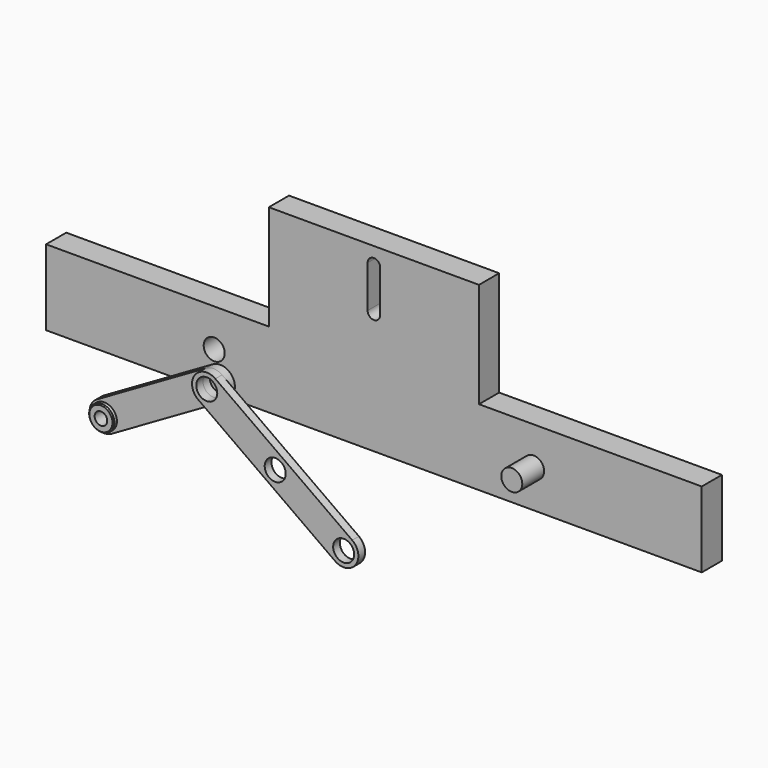
from build123d import *

# Parameters (mm, degrees)
F0_W      = 156
F0_H      = 6
F1_DEPTH  = 9
F2_R      = 2.5
F3_DEPTH  = 6
F5_R      = 2.5
F6_DEPTH  = 7
F7_R      = 2
F8_DEPTH  = 5
F9_R      = 2.5
F10_DEPTH = 6.5
F11_W     = 50
F11_H     = 6
F12_DEPTH = 25
F14_DEPTH = 6
F15_R     = 2.5
F16_DEPTH = 2
F17_R     = 2.5
F18_DEPTH = 2
F20_R     = 2.5
F21_DEPTH = 2.1
F22_R     = 3
F23_DEPTH = 1
F24_R     = 1.5
F25_DEPTH = 3.1
F26_SIZE  = 0.25


with BuildPart() as f1:
    # F0 (on Top) → F1 (new body, symmetric)
    with BuildSketch(Plane.XY):
        with Locations((0, -38.5)):
            Rectangle(F0_W, F0_H)
    extrude(amount=F1_DEPTH, both=True)

    # F2 (on face) → F3 (cut, through all)
    with BuildSketch(Plane.XZ.offset(41.5)):
        with Locations((-38, 0)):
            Circle(F2_R)
        with Locations((38, 0)):
            Circle(F2_R)
    extrude(amount=-F3_DEPTH, mode=Mode.SUBTRACT)

    # F11 (on face) → F12 (join)
    with BuildSketch(Plane.XY.offset(9)):
        with Locations((0, -38.5)):
            Rectangle(F11_W, F11_H)
    extrude(amount=F12_DEPTH)

    # F13 (on face) → F14 (cut, through all)
    with BuildSketch(Plane.XZ.offset(41.5)):
        with BuildLine():
            ThreePointArc((1.5, 30), (0, 31.5), (-1.5, 30))
            Line((-1.5, 30), (-1.5, 20))
            ThreePointArc((-1.5, 20), (0, 18.5), (1.5, 20))
            Line((1.5, 20), (1.5, 30))
        make_face()
    extrude(amount=-F14_DEPTH, mode=Mode.SUBTRACT)


with BuildPart() as f6:
    # F5 (on face) → F6 (new body)
    with BuildSketch(Plane.XZ.offset(41.5)):
        with Locations((38, 0)):
            Circle(F5_R)
    extrude(amount=-F6_DEPTH)

    # F7 (on face) → F8 (join)
    with BuildSketch(Plane(origin=(0, -34.5, 0), x_dir=(-1, 0, 0), z_dir=(0, 1, 0))):
        with Locations((-38, 0)):
            Circle(F7_R)
    extrude(amount=F8_DEPTH)

    # F9 (on face) → F10 (join)
    with BuildSketch(Plane.XZ.offset(41.5)):
        with Locations((38, 0)):
            Circle(F9_R)
    extrude(amount=F10_DEPTH)


with BuildPart() as f16:
    # F15 (on offset) → F16 (new body)
    with BuildSketch(Plane.XZ.offset(46.5)):
        with BuildLine():
            ThreePointArc((-60.3006148636, -14.8932962321), (-61.5817037769, -19.6743851453), (-56.8006148636, -20.9554740586))
            Line((-56.8006148636, -20.9554740586), (-30.8198527501, -5.9554740586))
            ThreePointArc((-30.8198527501, -5.9554740586), (-29.5387638369, -1.1743851453), (-34.3198527501, 0.1067037679))
            Line((-34.3198527501, 0.1067037679), (-60.3006148636, -14.8932962321))
        make_face()
        with Locations((-58.5506148636, -17.9243851453)):
            Circle(F15_R, mode=Mode.SUBTRACT)
        with Locations((-32.5698527501, -2.9243851453)):
            Circle(F15_R, mode=Mode.SUBTRACT)
    extrude(amount=F16_DEPTH)


with BuildPart() as f18:
    # F17 (on face) → F18 (new body)
    with BuildSketch(Plane.XZ.offset(48.5)):
        with BuildLine():
            ThreePointArc((-30.5382201412, -0.074390594), (-35.4198473014, -0.8927525364), (-34.601485359, -5.7743796966))
            Line((-34.601485359, -5.7743796966), (-2.0301190581, -28.9930380836))
            ThreePointArc((-2.0301190581, -28.9930380836), (2.8515081021, -28.1746761412), (2.0331461597, -23.293048981))
            Line((2.0331461597, -23.293048981), (-30.5382201412, -0.074390594))
        make_face()
        with Locations((0.0015135508, -26.1430435323)):
            Circle(F17_R, mode=Mode.SUBTRACT)
        with Locations((-32.5698527501, -2.9243851453)):
            Circle(F17_R, mode=Mode.SUBTRACT)
        with Locations((-16.2841695997, -14.5337143388)):
            Circle(F17_R, mode=Mode.SUBTRACT)
    extrude(amount=F18_DEPTH)


with BuildPart() as f21:
    # F20 (on face) → F21 (new body)
    with BuildSketch(Plane.XZ.offset(48.5)):
        with Locations((-58.5506148636, -17.9243851453)):
            Circle(F20_R)
    extrude(amount=-F21_DEPTH)

    # F22 (on face) → F23 (join)
    with BuildSketch(Plane.XZ.offset(48.5)):
        with Locations((-58.5506148636, -17.9243851453)):
            Circle(F22_R)
    extrude(amount=F23_DEPTH)

    # F24 (on face) → F25 (cut, through all)
    with BuildSketch(Plane.XZ.offset(49.5)):
        with Locations((-58.5506148636, -17.9243851453)):
            Circle(F24_R)
    extrude(amount=-F25_DEPTH, mode=Mode.SUBTRACT)

    # F26
    f26_edges = [f21.edges().sort_by_distance(p)[0] for p in [
        (-61.550615, -49.5, -17.924385),
        (-61.050615, -46.4, -17.924385),
    ]]
    chamfer(f26_edges, length=F26_SIZE)


solid = Compound([f1.part, f6.part, f16.part, f18.part, f21.part])
